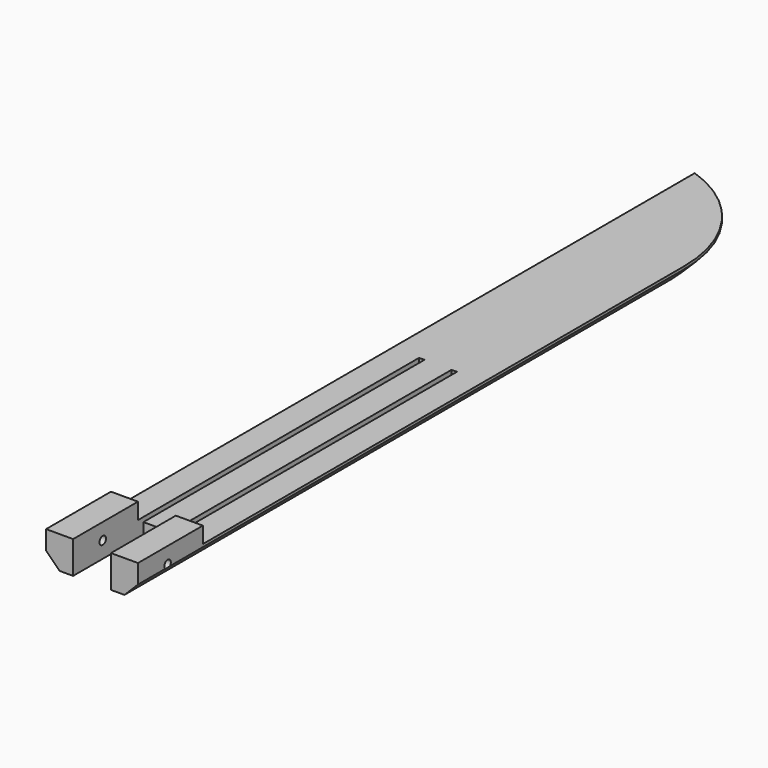
from build123d import *

# Parameters (mm, degrees)
F1_DEPTH    = 6
F2_W        = 10
F2_H        = 30
F3_DEPTH    = 6
F4_R        = 1.5
F5_DEPTH    = 34.001
F6_T1_DEPTH = 242.8543856465
F7_T1_DEPTH = 325.7168298797
F7_T3_DEPTH = 265.4875378105
F7_T6_ANGLE = 86.0754516161


# Not quite as in the source:
# - a fillet or chamfer that OpenCascade refuses, or shapes differently, is made with other operations: its cross-section is extruded or revolved along the edge and cut away or added


with BuildPart() as f1:
    # F0 (on Top) → F1 (new body)
    with BuildSketch(Plane.XY):
        Polygon((7, -150), (17, -150), (17, 150), (-17, 150), (-17, -150), (-7, -150), (-7, 10), (-5, 10), (-5, -120), (5, -120), (5, 10), (7, 10), align=None)
    extrude(amount=F1_DEPTH)

    # F2 (on face) → F3 (join)
    with BuildSketch(Plane.XY.offset(6)):
        with Locations((-12, -135)):
            Rectangle(F2_W, F2_H)
        with Locations((12, -135)):
            Rectangle(F2_W, F2_H)
    extrude(amount=F3_DEPTH)

    # F4 (on face) → F5 (cut, through all)
    with BuildSketch(Plane(origin=(-17, 0, 0), x_dir=(0, -1, 0), z_dir=(-1, 0, 0))):
        with Locations((136.3040655851, 6)):
            Circle(F4_R)
    extrude(amount=-F5_DEPTH, mode=Mode.SUBTRACT)

    # F6: fillet of radius 50 on 1 edges, made by hand

    # F6_s2 → F6_t1 (cut)
    with BuildSketch(Plane.XY.offset(-118.4271928233)):
        with BuildLine():
            ThreePointArc((17, 102.6291228707), (7.6201920232, 131.7838823449), (-17, 150))
            Line((-17, 150), (17, 150))
            Line((17, 150), (17, 102.6291228707))
        make_face()
    extrude(amount=F6_T1_DEPTH, mode=Mode.SUBTRACT)

    # F7: chamfer of 5 on 3 edges, made by hand

    # F7_s2 → F7_t1 (cut)
    with BuildSketch(Plane.XZ.offset(-162.8584149398)):
        Polygon((-12, 0), (-17, 5), (-17, 0), align=None)
    extrude(amount=F7_T1_DEPTH, mode=Mode.SUBTRACT)

    # F7_s4 → F7_t3 (cut)
    with BuildSketch(Plane.XZ.offset(-102.6291228707)):
        Polygon((17, 5), (12, 0), (17, 0), align=None)
    extrude(amount=F7_T3_DEPTH, mode=Mode.SUBTRACT)

    # F7_s5 → F7_t6 (revolve, cut)
    with BuildSketch(Plane(origin=(-39.8531616504, 2.7340709455, 0), x_dir=(0, 0, 1), z_dir=(-0.9976550461, 0.0684427424, 0))):
        Polygon((0, 145.1298518112), (5, 150.1298518112), (0, 150.1298518112), align=None)
    revolve(axis=Axis((-33, 102.6291228707, 0), (0, 0, -1)), revolution_arc=F7_T6_ANGLE, mode=Mode.SUBTRACT)


solid = f1.part
